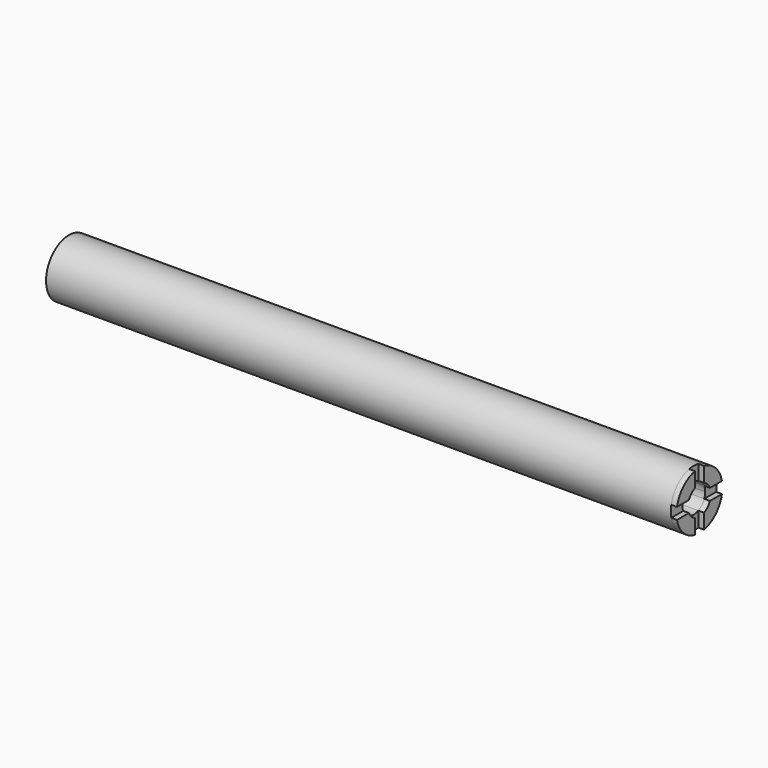
from build123d import *
from build123d import SkipClean  # not in build123d's __all__

# Parameters (mm, degrees)
F0_R     = 12.7
F1_DEPTH = 276.86
F3_DEPTH = 2.54
F4_DEPTH = 25.4


with BuildPart() as f1:
    # F0 (on Right) → F1 (new body)
    with BuildSketch(Plane.YZ):
        Circle(F0_R)
    extrude(amount=F1_DEPTH)

    # F2 (on face) → F3 (join)
    with BuildSketch(Plane.YZ.offset(276.86)):
        with BuildLine():
            ThreePointArc((2.54, 5.8198711326), (4.4901280605, 4.4901280605), (5.8198711326, 2.54))
            Line((5.8198711326, 2.54), (12.4434078933, 2.54))
            ThreePointArc((12.4434078933, 2.54), (8.9802561211, 8.9802561211), (2.54, 12.4434078933))
            Line((2.54, 12.4434078933), (2.54, 5.8198711326))
        make_face()
        with BuildLine():
            ThreePointArc((-5.8198711326, 2.54), (-4.4901280605, 4.4901280605), (-2.54, 5.8198711326))
            Line((-2.54, 5.8198711326), (-2.54, 12.4434078933))
            ThreePointArc((-2.54, 12.4434078933), (-8.9802561211, 8.9802561211), (-12.4434078933, 2.54))
            Line((-12.4434078933, 2.54), (-5.8198711326, 2.54))
        make_face()
        with BuildLine():
            Line((-2.54, -12.4434078933), (-2.54, -5.8198711326))
            ThreePointArc((-2.54, -5.8198711326), (-4.4901280605, -4.4901280605), (-5.8198711326, -2.54))
            Line((-5.8198711326, -2.54), (-12.4434078933, -2.54))
            ThreePointArc((-12.4434078933, -2.54), (-8.9802561211, -8.9802561211), (-2.54, -12.4434078933))
        make_face()
        with BuildLine():
            Line((12.4434078933, -2.54), (5.8198711326, -2.54))
            ThreePointArc((5.8198711326, -2.54), (4.4901280605, -4.4901280605), (2.54, -5.8198711326))
            Line((2.54, -5.8198711326), (2.54, -12.4434078933))
            ThreePointArc((2.54, -12.4434078933), (8.9802561211, -8.9802561211), (12.4434078933, -2.54))
        make_face()
    extrude(amount=F3_DEPTH)

    # F2 (on face) → F4 (cut)
    with BuildSketch(Plane.YZ.offset(276.86)):
        with BuildLine():
            ThreePointArc((5.8198711326, -2.54), (6.2160550871, -1.2973662374), (6.35, 0))
            ThreePointArc((6.35, 0), (6.2160550871, 1.2973662374), (5.8198711326, 2.54))
            ThreePointArc((5.8198711326, 2.54), (4.4901280605, 4.4901280605), (2.54, 5.8198711326))
            ThreePointArc((2.54, 5.8198711326), (0, 6.35), (-2.54, 5.8198711326))
            ThreePointArc((-2.54, 5.8198711326), (-4.4901280605, 4.4901280605), (-5.8198711326, 2.54))
            ThreePointArc((-5.8198711326, 2.54), (-6.35, 0), (-5.8198711326, -2.54))
            ThreePointArc((-5.8198711326, -2.54), (-4.4901280605, -4.4901280605), (-2.54, -5.8198711326))
            ThreePointArc((-2.54, -5.8198711326), (0, -6.35), (2.54, -5.8198711326))
            ThreePointArc((2.54, -5.8198711326), (4.4901280605, -4.4901280605), (5.8198711326, -2.54))
        make_face()
    with SkipClean():  # cleaning this boolean's faces spoils the solid; the shape is the same uncleaned
        extrude(amount=-F4_DEPTH, mode=Mode.SUBTRACT)


solid = f1.part
